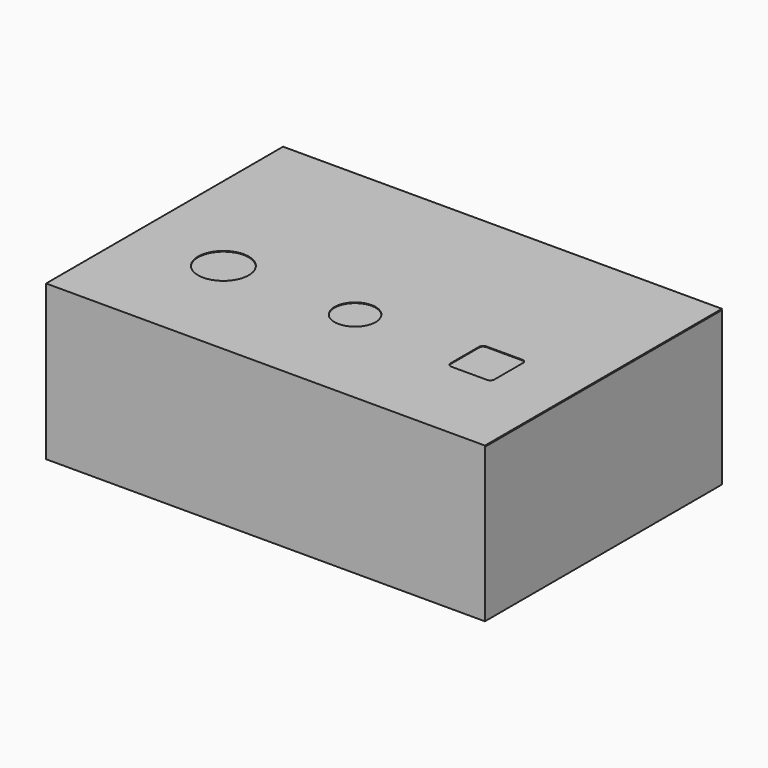
from build123d import *

# Parameters (mm, degrees)
F1_DEPTH = 127
F3_DEPTH = 0.4064


# Not quite as in the source:
# - the dataset's text gives a spline's control points without its knots; the knots are read off the source's solid


with BuildPart() as f1:
    # F0 (on Right) → F1 (new body, symmetric)
    with BuildSketch(Plane.YZ):
        Polygon((-171.45, 0), (0, 0), (0, 88.9), (-171.0436, 88.9), (-171.0436, 89.154), (0, 89.154), (0, 89.5604), (-171.45, 89.5604), align=None)
    extrude(amount=F1_DEPTH, both=True)

    # F2 (on face) → F3 (cut, through all)
    with BuildSketch(Plane.XY.offset(89.5604)):
        with BuildLine():
            add(Edge.make_bspline(
                [(89.2501661772, -119.9617381969), (89.6911355772, -119.5207687969), (89.9481327772, -118.9020247969), (89.9481327772, -118.2782769969)],
                knots=[1, 1, 1, 1, 2, 2, 2, 2], degree=3))
            Line((89.9481327772, -118.2782769969), (89.9481327772, -97.6407769969))
            add(Edge.make_bspline(
                [(89.9481327772, -97.6407769969), (89.9481327772, -97.0166989969), (89.6911355772, -96.3979803969), (89.2501661772, -95.9570109969)],
                knots=[0, 0, 0, 0, 1, 1, 1, 1], degree=3))
            add(Edge.make_bspline(
                [(89.2501661772, -95.9570109969), (88.8091967772, -95.5160161969), (88.1904527772, -95.2595269969), (87.5668827772, -95.2595269969)],
                knots=[1, 1, 1, 1, 2, 2, 2, 2], degree=3))
            Line((87.5668827772, -95.2595269969), (66.9293827772, -95.2595269969))
            add(Edge.make_bspline(
                [(66.9293827772, -95.2595269969), (66.3058127772, -95.2595269969), (65.6863829772, -95.5160161969), (65.2457691772, -95.9570109969)],
                knots=[0, 0, 0, 0, 1, 1, 1, 1], degree=3))
            add(Edge.make_bspline(
                [(65.2457691772, -95.9570109969), (64.8051299772, -96.3979803969), (64.5481327772, -97.0166989969), (64.5481327772, -97.6407769969)],
                knots=[1, 1, 1, 1, 2, 2, 2, 2], degree=3))
            Line((64.5481327772, -97.6407769969), (64.5481327772, -118.2782769969))
            add(Edge.make_bspline(
                [(64.5481327772, -118.2782769969), (64.5481327772, -118.9020247969), (64.8051299772, -119.5207687969), (65.2457691772, -119.9617381969)],
                knots=[0, 0, 0, 0, 1, 1, 1, 1], degree=3))
            add(Edge.make_bspline(
                [(65.2457691772, -119.9617381969), (65.6863829772, -120.4023519969), (66.3058127772, -120.6595269969), (66.9293827772, -120.6595269969)],
                knots=[1, 1, 1, 1, 2, 2, 2, 2], degree=3))
            Line((66.9293827772, -120.6595269969), (87.5668827772, -120.6595269969))
            add(Edge.make_bspline(
                [(87.5668827772, -120.6595269969), (88.1904527772, -120.6595269969), (88.8091967772, -120.4023519969), (89.2501661772, -119.9617381969)],
                knots=[0, 0, 0, 0, 1, 1, 1, 1], degree=3))
        make_face()
        with BuildLine():
            add(Edge.make_bspline(
                [(-64.7683472228, -97.5754989969), (-67.4865282228, -94.8573179969), (-71.3078058228, -93.2749995969), (-75.1518672228, -93.2749995969)],
                knots=[7, 7, 7, 7, 8, 8, 8, 8], degree=3))
            add(Edge.make_bspline(
                [(-75.1518672228, -93.2749995969), (-78.9959032228, -93.2749995969), (-82.8171808228, -94.8573179969), (-85.5353872228, -97.5754989969)],
                knots=[0, 0, 0, 0, 1, 1, 1, 1], degree=3))
            add(Edge.make_bspline(
                [(-85.5353872228, -97.5754989969), (-88.2542286228, -100.2940101969), (-89.8362422228, -104.1149829969), (-89.8362422228, -107.9595269969), (-89.8362422228, -111.8033851969), (-88.2542286228, -115.6243579969), (-85.5353872228, -118.3425389969)],
                knots=[1, 1, 1, 1, 2, 2, 2, 3, 3, 3, 3], degree=3))
            add(Edge.make_bspline(
                [(-85.5353872228, -118.3425389969), (-82.8171808228, -121.0614057969), (-78.9959032228, -122.6440797969), (-75.1518672228, -122.6440797969), (-71.3078058228, -122.6440797969), (-67.4865282228, -121.0614057969), (-64.7683472228, -118.3425389969)],
                knots=[3, 3, 3, 3, 4, 4, 4, 5, 5, 5, 5], degree=3))
            add(Edge.make_bspline(
                [(-64.7683472228, -118.3425389969), (-62.0501408228, -115.6243579969), (-60.4674922228, -111.8033851969), (-60.4674922228, -107.9595269969), (-60.4674922228, -104.1149829969), (-62.0501408228, -100.2940101969), (-64.7683472228, -97.5754989969)],
                knots=[5, 5, 5, 5, 6, 6, 6, 7, 7, 7, 7], degree=3))
        make_face()
        with BuildLine():
            add(Edge.make_bspline(
                [(9.4669119772, -99.5405953969), (7.2627507772, -97.3364087969), (4.1656017772, -96.0532769969), (1.0484883772, -96.0532769969)],
                knots=[7, 7, 7, 7, 8, 8, 8, 8], degree=3))
            add(Edge.make_bspline(
                [(1.0484883772, -96.0532769969), (-2.0690060228, -96.0532769969), (-5.1664598228, -97.3364087969), (-7.3706464228, -99.5405953969)],
                knots=[0, 0, 0, 0, 1, 1, 1, 1], degree=3))
            add(Edge.make_bspline(
                [(-7.3706464228, -99.5405953969), (-9.5748076228, -101.7447311969), (-10.8577616228, -104.8424135969), (-10.8577616228, -107.9595269969), (-10.8577616228, -111.0768435969), (-9.5748076228, -114.1744751969), (-7.3706464228, -116.3774679969)],
                knots=[1, 1, 1, 1, 2, 2, 2, 3, 3, 3, 3], degree=3))
            add(Edge.make_bspline(
                [(-7.3706464228, -116.3774679969), (-5.1664598228, -118.5816291969), (-2.0690060228, -119.8657769969), (1.0484883772, -119.8657769969), (4.1656017772, -119.8657769969), (7.2627507772, -118.5816291969), (9.4669119772, -116.3774679969)],
                knots=[3, 3, 3, 3, 4, 4, 4, 5, 5, 5, 5], degree=3))
            add(Edge.make_bspline(
                [(9.4669119772, -116.3774679969), (11.6710985772, -114.1744751969), (12.9547383772, -111.0768435969), (12.9547383772, -107.9595269969), (12.9547383772, -104.8424135969), (11.6710985772, -101.7447311969), (9.4669119772, -99.5405953969)],
                knots=[5, 5, 5, 5, 6, 6, 6, 7, 7, 7, 7], degree=3))
        make_face()
    extrude(amount=-F3_DEPTH, mode=Mode.SUBTRACT)


solid = f1.part
